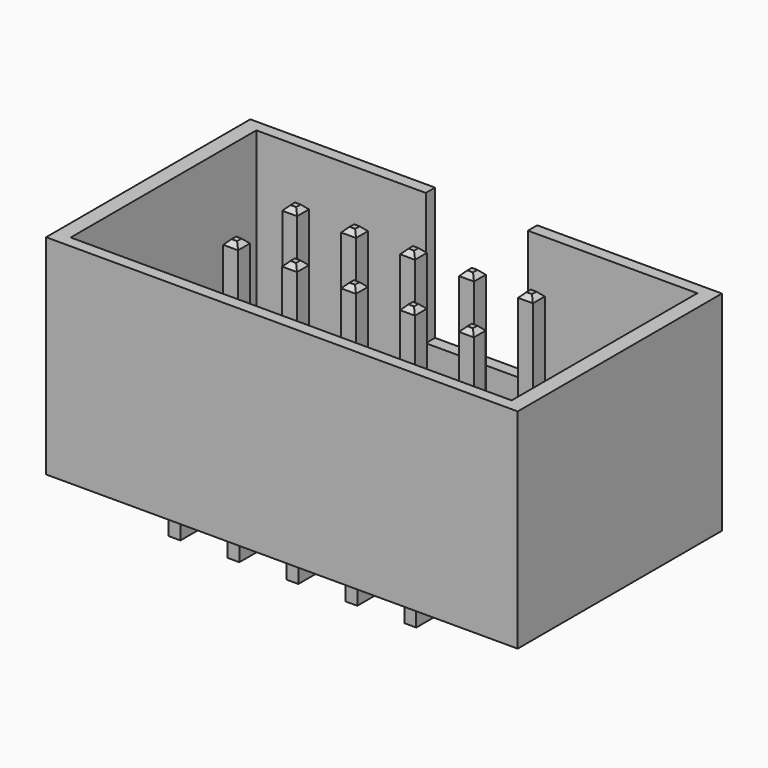
from build123d import *

# Parameters (mm, degrees)
F0_W       = 20.32
F0_H       = 11
F0_W_2     = 19
F0_H_2     = 10
F1_DEPTH   = 9
F0_W_3     = 0.64
F0_H_3     = 0.64
F2_DEPTH   = 1
F3_DEPTH   = 9
F4_SIZE    = 0.2
F4_2_SIZE  = 0.2
F4_3_SIZE  = 0.2
F4_4_SIZE  = 0.2
F4_5_SIZE  = 0.2
F4_6_SIZE  = 0.2
F6_W       = 4.4
F6_H       = 0.5
F7_DEPTH   = 5.7
F9_W       = 0.5111949686
F9_H       = 3.9092235888
F10_DEPTH  = 1
F11_DEPTH  = 9
F12_SIZE   = 0.2
F12_2_SIZE = 0.2
F12_3_SIZE = 0.2
F12_4_SIZE = 0.2


# Not quite as in the source:
# - a feature names something its author has since deleted; it is built from what else it names


with BuildPart() as f1:
    # F0 (on Top) → F1 (new body)
    with BuildSketch(Plane.XY):
        Rectangle(F0_W, F0_H)
        Rectangle(F0_W_2, F0_H_2, mode=Mode.SUBTRACT)
    extrude(amount=F1_DEPTH)

    # F0 (on Top) → F2 (join)
    with BuildSketch(Plane.XY):
        Rectangle(F0_W_2, F0_H_2)
        with Locations((-5.08, -1.59)):
            Rectangle(F0_W_3, F0_H_3, mode=Mode.SUBTRACT)
        with Locations((-2.54, -1.59)):
            Rectangle(F0_W_3, F0_H_3, mode=Mode.SUBTRACT)
        with Locations((0, -1.59)):
            Rectangle(F0_W_3, F0_H_3, mode=Mode.SUBTRACT)
        with Locations((2.54, -1.59)):
            Rectangle(F0_W_3, F0_H_3, mode=Mode.SUBTRACT)
        with Locations((5.08, -1.59)):
            Rectangle(F0_W_3, F0_H_3, mode=Mode.SUBTRACT)
        with Locations((-5.08, 1.59)):
            Rectangle(F0_W_3, F0_H_3, mode=Mode.SUBTRACT)
        with Locations((-2.54, 1.59)):
            Rectangle(F0_W_3, F0_H_3, mode=Mode.SUBTRACT)
        with Locations((0, 1.59)):
            Rectangle(F0_W_3, F0_H_3, mode=Mode.SUBTRACT)
        with Locations((2.54, 1.59)):
            Rectangle(F0_W_3, F0_H_3, mode=Mode.SUBTRACT)
        with Locations((5.08, 1.59)):
            Rectangle(F0_W_3, F0_H_3, mode=Mode.SUBTRACT)
    extrude(amount=F2_DEPTH)

    # F6 (on offset) → F7 (cut)
    with BuildSketch(Plane.XY.offset(3.3)):
        with Locations((0, 5.25)):
            Rectangle(F6_W, F6_H)
    extrude(amount=F7_DEPTH, mode=Mode.SUBTRACT)


with BuildPart() as f3:
    # F0 (on Top) → F3 (new body)
    with BuildSketch(Plane.XY):
        with Locations((0, -1.59)):
            Rectangle(F0_W_3, F0_H_3)
    extrude(amount=F3_DEPTH)

    # F4#2
    f4_2_edges = [f3.edges().sort_by_distance(p)[0] for p in [
        (0, -1.27, 9),
        (-0.32, -1.59, 9),
        (0, -1.91, 9),
        (0.32, -1.59, 9),
    ]]
    chamfer(f4_2_edges, length=F4_2_SIZE)


with BuildPart() as f3b:
    # F0 (on Top) → F3, piece 2 (new body)
    with BuildSketch(Plane.XY):
        with Locations((0, 1.59)):
            Rectangle(F0_W_3, F0_H_3)
    extrude(amount=F3_DEPTH)

    # F4
    f4_edges = [f3b.edges().sort_by_distance(p)[0] for p in [
        (-0.32, 1.59, 9),
        (0, 1.27, 9),
        (0.32, 1.59, 9),
        (0, 1.91, 9),
    ]]
    chamfer(f4_edges, length=F4_SIZE)


with BuildPart() as f3c:
    # F0 (on Top) → F3, piece 3 (new body)
    with BuildSketch(Plane.XY):
        with Locations((2.54, 1.59)):
            Rectangle(F0_W_3, F0_H_3)
    extrude(amount=F3_DEPTH)

    # F4#4
    f4_4_edges = [f3c.edges().sort_by_distance(p)[0] for p in [
        (2.22, 1.59, 9),
        (2.54, 1.27, 9),
        (2.86, 1.59, 9),
        (2.54, 1.91, 9),
    ]]
    chamfer(f4_4_edges, length=F4_4_SIZE)


with BuildPart() as f3d:
    # F0 (on Top) → F3, piece 4 (new body)
    with BuildSketch(Plane.XY):
        with Locations((2.54, -1.59)):
            Rectangle(F0_W_3, F0_H_3)
    extrude(amount=F3_DEPTH)

    # F4#3
    f4_3_edges = [f3d.edges().sort_by_distance(p)[0] for p in [
        (2.22, -1.59, 9),
        (2.54, -1.91, 9),
        (2.86, -1.59, 9),
        (2.54, -1.27, 9),
    ]]
    chamfer(f4_3_edges, length=F4_3_SIZE)


with BuildPart() as f3e:
    # F0 (on Top) → F3, piece 5 (new body)
    with BuildSketch(Plane.XY):
        with Locations((5.08, 1.59)):
            Rectangle(F0_W_3, F0_H_3)
    extrude(amount=F3_DEPTH)

    # F4#5
    f4_5_edges = [f3e.edges().sort_by_distance(p)[0] for p in [
        (4.76, 1.59, 9),
        (5.08, 1.27, 9),
        (5.08, 1.91, 9),
        (5.4, 1.59, 9),
    ]]
    chamfer(f4_5_edges, length=F4_5_SIZE)


with BuildPart() as f3f:
    # F0 (on Top) → F3, piece 6 (new body)
    with BuildSketch(Plane.XY):
        with Locations((5.08, -1.59)):
            Rectangle(F0_W_3, F0_H_3)
    extrude(amount=F3_DEPTH)

    # F4#6
    f4_6_edges = [f3f.edges().sort_by_distance(p)[0] for p in [
        (5.08, -1.27, 9),
        (4.76, -1.59, 9),
        (5.08, -1.91, 9),
        (5.4, -1.59, 9),
    ]]
    chamfer(f4_6_edges, length=F4_6_SIZE)


with BuildPart() as f10:
    # F9 (on offset) → F10 (new body)
    with BuildSketch(Plane.XY.offset(-1)):
        with Locations((5.0781009255, -2.9758856997)):
            Rectangle(F9_W, F9_H)
    extrude(amount=F10_DEPTH)


with BuildPart() as f10b:
    # F9 (on offset) → F10, piece 2 (new body)
    with BuildSketch(Plane.XY.offset(-1)):
        with Locations((2.5381009255, -2.9758856997)):
            Rectangle(F9_W, F9_H)
    extrude(amount=F10_DEPTH)


with BuildPart() as f10c:
    # F9 (on offset) → F10, piece 3 (new body)
    with BuildSketch(Plane.XY.offset(-1)):
        with Locations((-0.0018990745, -2.9758856997)):
            Rectangle(F9_W, F9_H)
    extrude(amount=F10_DEPTH)


with BuildPart() as f10d:
    # F9 (on offset) → F10, piece 4 (new body)
    with BuildSketch(Plane.XY.offset(-1)):
        with Locations((-2.5418990745, -2.9758856997)):
            Rectangle(F9_W, F9_H)
    extrude(amount=F10_DEPTH)


with BuildPart() as f10e:
    # F9 (on offset) → F10, piece 5 (new body)
    with BuildSketch(Plane.XY.offset(-1)):
        with Locations((-5.0818990745, -2.9758856997)):
            Rectangle(F9_W, F9_H)
    extrude(amount=F10_DEPTH)


with BuildPart() as f10f:
    # F9 (on offset) → F10, piece 6 (new body)
    with BuildSketch(Plane.XY.offset(-1)):
        with Locations((-5.0818990745, 2.9747432311)):
            Rectangle(F9_W, F9_H)
    extrude(amount=F10_DEPTH)


with BuildPart() as f10g:
    # F9 (on offset) → F10, piece 7 (new body)
    with BuildSketch(Plane.XY.offset(-1)):
        with Locations((-2.5418990745, 2.9747432311)):
            Rectangle(F9_W, F9_H)
    extrude(amount=F10_DEPTH)


with BuildPart() as f10h:
    # F9 (on offset) → F10, piece 8 (new body)
    with BuildSketch(Plane.XY.offset(-1)):
        with Locations((-0.0018990745, 2.9747432311)):
            Rectangle(F9_W, F9_H)
    extrude(amount=F10_DEPTH)


with BuildPart() as f10i:
    # F9 (on offset) → F10, piece 9 (new body)
    with BuildSketch(Plane.XY.offset(-1)):
        with Locations((2.5381009255, 2.9747432311)):
            Rectangle(F9_W, F9_H)
    extrude(amount=F10_DEPTH)


with BuildPart() as f10j:
    # F9 (on offset) → F10, piece 10 (new body)
    with BuildSketch(Plane.XY.offset(-1)):
        with Locations((5.0781009255, 2.9747432311)):
            Rectangle(F9_W, F9_H)
    extrude(amount=F10_DEPTH)


with BuildPart() as f11:
    # F0 (on Top) → F11 (new body)
    with BuildSketch(Plane.XY):
        with Locations((-5.08, 1.59)):
            Rectangle(F0_W_3, F0_H_3)
    extrude(amount=F11_DEPTH)

    # F12
    f12_edges = [f11.edges().sort_by_distance(p)[0] for p in [
        (-5.4, 1.59, 9),
        (-5.08, 1.91, 9),
        (-5.08, 1.27, 9),
        (-4.76, 1.59, 9),
    ]]
    chamfer(f12_edges, length=F12_SIZE)


with BuildPart() as f11b:
    # F0 (on Top) → F11, piece 2 (new body)
    with BuildSketch(Plane.XY):
        with Locations((-2.54, 1.59)):
            Rectangle(F0_W_3, F0_H_3)
    extrude(amount=F11_DEPTH)

    # F12#2
    f12_2_edges = [f11b.edges().sort_by_distance(p)[0] for p in [
        (-2.86, 1.59, 9),
        (-2.54, 1.91, 9),
        (-2.22, 1.59, 9),
        (-2.54, 1.27, 9),
    ]]
    chamfer(f12_2_edges, length=F12_2_SIZE)


with BuildPart() as f11c:
    # F0 (on Top) → F11, piece 3 (new body)
    with BuildSketch(Plane.XY):
        with Locations((-2.54, -1.59)):
            Rectangle(F0_W_3, F0_H_3)
    extrude(amount=F11_DEPTH)

    # F12#4
    f12_4_edges = [f11c.edges().sort_by_distance(p)[0] for p in [
        (-2.86, -1.59, 9),
        (-2.54, -1.91, 9),
        (-2.22, -1.59, 9),
        (-2.54, -1.27, 9),
    ]]
    chamfer(f12_4_edges, length=F12_4_SIZE)


with BuildPart() as f11d:
    # F0 (on Top) → F11, piece 4 (new body)
    with BuildSketch(Plane.XY):
        with Locations((-5.08, -1.59)):
            Rectangle(F0_W_3, F0_H_3)
    extrude(amount=F11_DEPTH)

    # F12#3
    f12_3_edges = [f11d.edges().sort_by_distance(p)[0] for p in [
        (-5.4, -1.59, 9),
        (-5.08, -1.27, 9),
        (-4.76, -1.59, 9),
        (-5.08, -1.91, 9),
    ]]
    chamfer(f12_3_edges, length=F12_3_SIZE)


solid = Compound([f1.part, f3.part, f3b.part, f3c.part, f3d.part, f3e.part, f3f.part, f10.part, f10b.part, f10c.part, f10d.part, f10e.part, f10f.part, f10g.part, f10h.part, f10i.part, f10j.part, f11.part, f11b.part, f11c.part, f11d.part])
